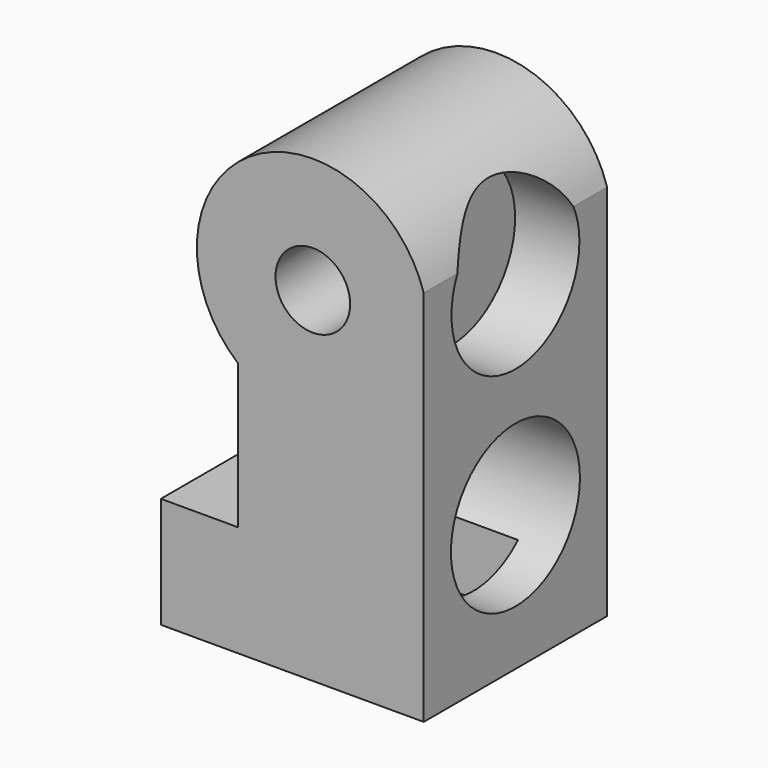
from build123d import *

# Parameters (mm, degrees)
F0_R      = 3.48
F1_DEPTH  = 6.88
F2_R      = 1.12
F3_DEPTH  = 6.23
F5_DEPTH  = 25
F7_DEPTH  = 6.88
F8_W      = 5.37
F8_H      = 4.36
F9_DEPTH  = 2.32
F10_R     = 2.4
F11_DEPTH = 1.93
F12_R     = 2.42
F13_DEPTH = 4.99


# Not quite as in the source:
# - a feature names something its author has since deleted; it is built from what else it names


with BuildPart() as f1:
    # F0 (on Front) → F1 (new body)
    with BuildSketch(Plane.XZ):
        Circle(F0_R)
    extrude(amount=F1_DEPTH)

    # F2 (on face) → F3 (cut)
    with BuildSketch(Plane.XZ.offset(6.88)):
        Circle(F2_R)
    extrude(amount=-F3_DEPTH, mode=Mode.SUBTRACT)

    # F4 (on face) → F5 (cut)
    with BuildSketch(Plane.XZ.offset(6.88)):
        Polygon((7.0880088024, -1.4447768917), (3.33, 4.3651785166), (3.33, -5.8573421486), align=None)
    extrude(amount=-F5_DEPTH, mode=Mode.SUBTRACT)

    # F6 (on face) → F7 (join)
    with BuildSketch(Plane.XZ.offset(6.88)):
        with BuildLine():
            Line((3.33, -10.3206928317), (3.33, -1.0106928317))
            ThreePointArc((3.33, -1.0106928317), (0.8809060484, -2.9691576427), (-2.24, -2.6632311203))
            Line((-2.24, -2.6632311203), (-2.24, -6.9906928317))
            Line((-2.24, -6.9906928317), (-4.56, -6.9906928317))
            Line((-4.56, -6.9906928317), (-4.56, -10.3206928317))
            Line((-4.56, -10.3206928317), (3.33, -10.3206928317))
        make_face()
    extrude(amount=-F7_DEPTH)

    # F8 (on face) → F9 (cut)
    with BuildSketch(Plane(origin=(0, 0, -10.3206928317), x_dir=(1, 0, 0), z_dir=(0, 0, -1))):
        with Locations((-0.615, 3.44)):
            Rectangle(F8_W, F8_H)
    extrude(amount=-F9_DEPTH, mode=Mode.SUBTRACT)

    # F10 (on face) → F11 (cut)
    with BuildSketch(Plane.YZ.offset(3.33)):
        with Locations((-3.44, 0)):
            Circle(F10_R)
    extrude(amount=-F11_DEPTH, mode=Mode.SUBTRACT)

    # F12 (on face) → F13 (cut)
    with BuildSketch(Plane.YZ.offset(3.33)):
        with Locations((-3.44, -6.2506928317)):
            Circle(F12_R)
    extrude(amount=-F13_DEPTH, mode=Mode.SUBTRACT)


solid = f1.part
